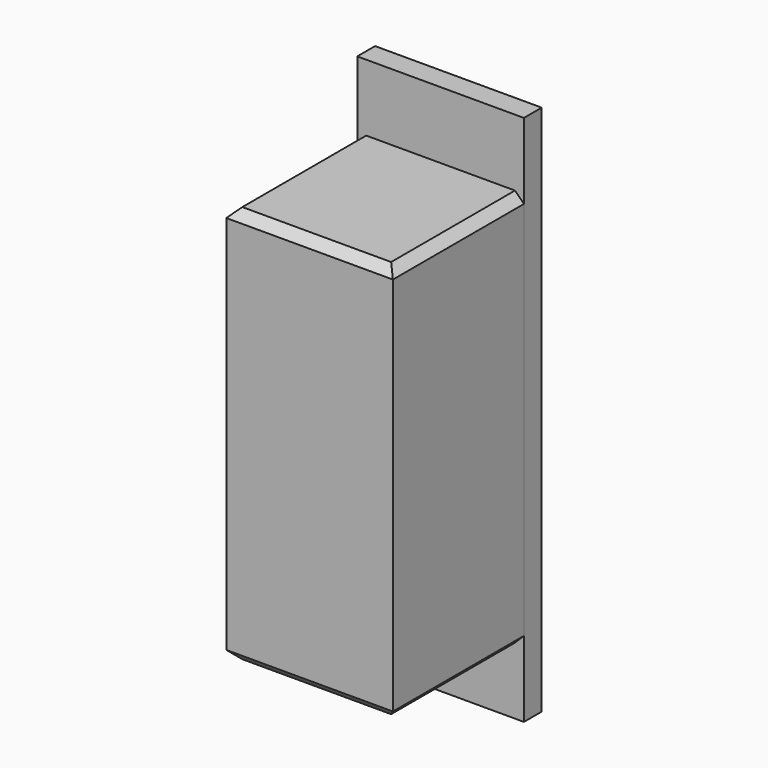
from build123d import *

# Parameters (mm, degrees)
F0_W     = 189.992
F0_H     = 453.898
F1_DEPTH = 212.09
F2_SIZE  = 10.16
F3_SIZE  = 10.16
F0_H_2   = 76.2
F4_DEPTH = 25.4


with BuildPart() as f1:
    # F0 (on Front) → F1 (new body)
    with BuildSketch(Plane.XZ):
        with Locations((94.996, -226.949)):
            Rectangle(F0_W, F0_H)
    extrude(amount=F1_DEPTH)

    # F2
    f2_edges = [f1.edges().sort_by_distance(p)[0] for p in [
        (0, -106.045, 0),
        (189.992, -106.045, 0),
        (189.992, -106.045, -453.898),
        (0, -106.045, -453.898),
    ]]
    chamfer(f2_edges, length=F2_SIZE)

    # F3
    f3_edges = [f1.edges().sort_by_distance(p)[0] for p in [
        (94.996, -212.09, 0),
        (94.996, -212.09, -453.898),
    ]]
    chamfer(f3_edges, length=F3_SIZE)


with BuildPart() as f4:
    # F0 (on Front) → F4 (new body)
    with BuildSketch(Plane.XZ):
        with Locations((94.996, 38.1)):
            Rectangle(F0_W, F0_H_2)
        with Locations((94.996, -491.998)):
            Rectangle(F0_W, F0_H_2)
        with Locations((94.996, -226.949)):
            Rectangle(F0_W, F0_H)
    extrude(amount=F4_DEPTH)


solid = Compound([f1.part, f4.part])
